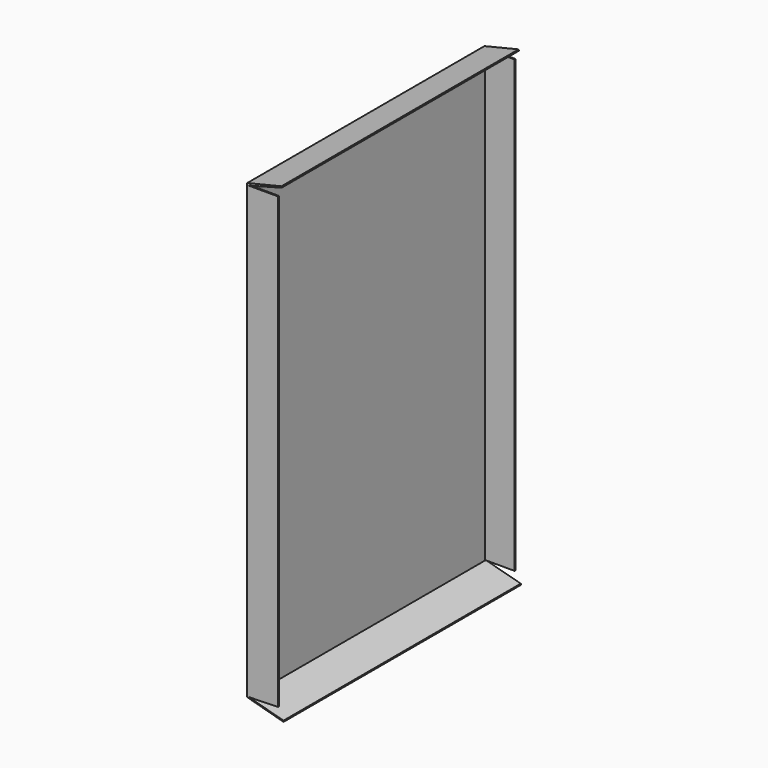
from build123d import *

# Parameters (mm, degrees)
F1_DEPTH = 247
F2_W     = 25
F2_H     = 1
F3_DEPTH = 1
F2_H_2   = 374
F4_DEPTH = 1
F6_DEPTH = 1


# Not quite as in the source:
# - a feature names something its author has since deleted; it is built from what else it names


with BuildPart() as f1:
    # F0 (on Front) → F1 (new body)
    with BuildSketch(Plane.XZ):
        Polygon((-1.1216281516, 73.3666580543), (-1.1216281516, 72.3666580543), (-1.1216281516, -302.6333419457), (-1.1216281516, -303.6333419457), (29.1284304133, -311.9432493216), (29.1284304133, -310.9432493216), (0, -303.1383099156), (0, 71.8616900844), (27.561313438, 79.2467217624), (27.3271471585, 80.2189183236), align=None)
    extrude(amount=F1_DEPTH)

    # F2 (on Front) → F3 (join)
    with BuildSketch(Plane.XZ):
        with Locations((12.390091487, 71.8666580543)):
            Rectangle(F2_W, F2_H)
    extrude(amount=F3_DEPTH)

    # F2 (on Front) → F4 (join)
    with BuildSketch(Plane.XZ):
        with Locations((12.390091487, -115.6333419457)):
            Rectangle(F2_W, F2_H_2)
    extrude(amount=F4_DEPTH)

    # F5 (on face) → F6 (join)
    with BuildSketch(Plane.XZ.offset(247)):
        Polygon((24.5685894042, 71.8616900844), (0, 71.8616900844), (0, -303.1383099156), (24.5685894042, -302.4606704712), align=None)
    extrude(amount=-F6_DEPTH)


solid = f1.part
